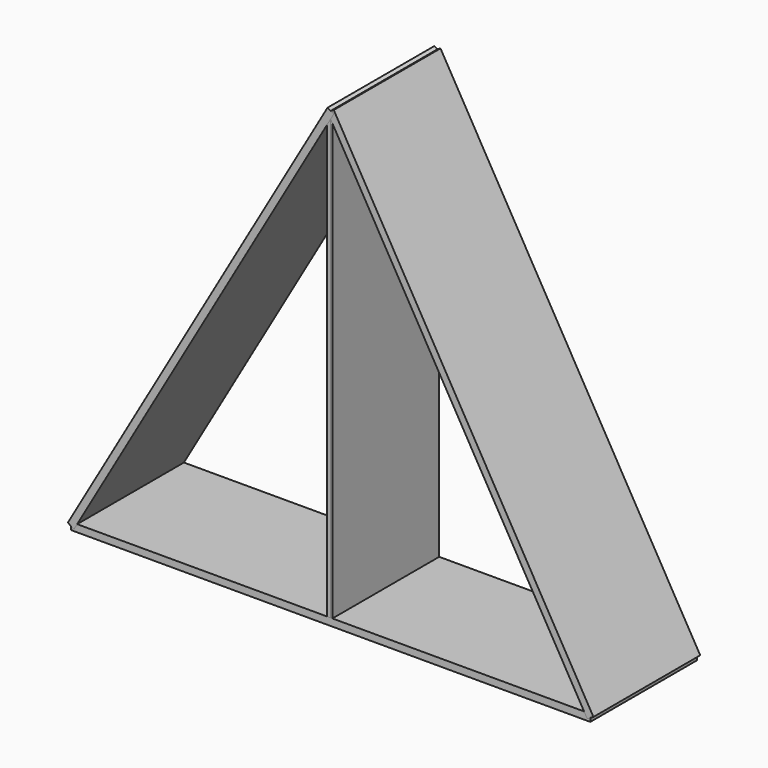
from build123d import *

# Parameters (mm, degrees)
F2_E1_W  = 791.8936292205
F2_E1_H  = 234.95
F3_DEPTH = 3.175
F1_E0_W  = 914.4
F1_E0_H  = 234.95
F5_DEPTH = 6.35
F1_E3_W  = 914.4
F1_E3_H  = 234.95
F6_DEPTH = 6.35
F1_E2_W  = 914.4
F1_E2_H  = 234.95
F7_DEPTH = 6.35


# Not quite as in the source:
# - a feature of the source that left no trace in its solid (it failed there, or was rolled back) is left out
# - a pattern or mirror of a feature is missing from the dataset's text; its kind, count and spacing are read off the source's solid
# - the program builds the solid bodies; features that only make, move or delete a surface that nothing else refers to are left out


with BuildPart() as f3:
    # F2_E1 (on explicit) → F3 (new body, symmetric)
    with BuildSketch(Plane(origin=(0, 0, -84.7172419105), x_dir=(0, 0, 1), z_dir=(1, 0, 0))):
        with Locations((395.9468146102, 117.475)):
            Rectangle(F2_E1_W, F2_E1_H)
    extrude(amount=F3_DEPTH, both=True)


with BuildPart() as f3_copies_1:
    # F3_copies: instance of F3
    add(f3.part.mirror(Plane(origin=(-1.5875, 0, 0), x_dir=(0, 0, -1), z_dir=(-1, 0, 0))))


with BuildPart() as f5:
    # F1_E0 (on explicit) → F5 (new body, symmetric)
    with BuildSketch(Plane(origin=(457.2, 0, -84.7172419105), x_dir=(-1, 0, 0), z_dir=(0, 0, 1))):
        with Locations((457.2, 117.475)):
            Rectangle(F1_E0_W, F1_E0_H)
    extrude(amount=F5_DEPTH, both=True)


with BuildPart() as f6:
    # F1_E3 (on explicit) → F6 (new body, symmetric)
    with BuildSketch(Plane(origin=(457.2, 0, -84.7172419105), x_dir=(-0.5, 0, 0.8660254038), z_dir=(0.8660254038, 0, 0.5))):
        with Locations((457.2, 117.475)):
            Rectangle(F1_E3_W, F1_E3_H)
    extrude(amount=F6_DEPTH, both=True)


with BuildPart() as f7:
    # F1_E2 (on explicit) → F7 (new body, symmetric)
    with BuildSketch(Plane(origin=(0, 0, 707.17638731), x_dir=(-0.5, 0, -0.8660254038), z_dir=(-0.8660254038, 0, 0.5))):
        with Locations((457.2, 117.475)):
            Rectangle(F1_E2_W, F1_E2_H)
    extrude(amount=F7_DEPTH, both=True)


solid = Compound([f3.part, f3_copies_1.part, f5.part, f6.part, f7.part])
